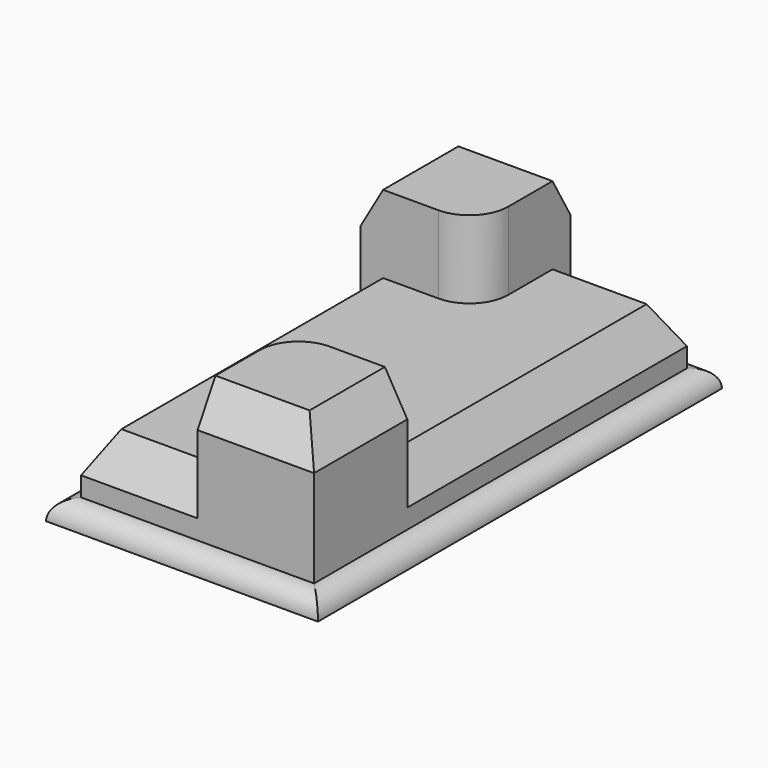
from build123d import *

# Parameters (mm, degrees)
F0_W     = 88.9
F0_H     = 165.1
F1_DEPTH = 6.35
F2_DEPTH = 25.4
F3_DEPTH = 50.8
F4_R     = 6.34999
F5_SIZE2 = 7.3323484187
F5_SIZE  = 12.7
F6_SIZE2 = 7.3323484187
F6_SIZE  = 12.7


# Not quite as in the source:
# - a fillet or chamfer is up to 0.001 mm smaller than in the source, because OpenCascade refuses the exact size


with BuildPart() as f1:
    # F0 (on Top) → F1 (new body)
    with BuildSketch(Plane.XY):
        Rectangle(F0_W, F0_H)
        Polygon((0, 76.2), (38.1, 76.2), (38.1, -38.1), (38.1, -76.2), (0, -76.2), (-38.1, -76.2), (-38.1, 38.1), (-38.1, 76.2), align=None, mode=Mode.SUBTRACT)
    extrude(amount=F1_DEPTH)

    # F0 (on Top) → F2 (join)
    with BuildSketch(Plane.XY):
        with BuildLine():
            Line((38.1, -38.1), (38.1, 76.2))
            Line((38.1, 76.2), (0, 76.2))
            Line((0, 76.2), (0, 50.8))
            ThreePointArc((0, 50.8), (-3.7197438789, 41.8197438789), (-12.7, 38.1))
            Line((-12.7, 38.1), (-38.1, 38.1))
            Line((-38.1, 38.1), (-38.1, -76.2))
            Line((-38.1, -76.2), (0, -76.2))
            Line((0, -76.2), (0, -50.8))
            ThreePointArc((0, -50.8), (3.7197438789, -41.8197438789), (12.7, -38.1))
            Line((12.7, -38.1), (38.1, -38.1))
        make_face()
    extrude(amount=F2_DEPTH)

    # F0 (on Top) → F3 (join)
    with BuildSketch(Plane.XY):
        with BuildLine():
            Line((0, 50.8), (0, 76.2))
            Line((0, 76.2), (-38.1, 76.2))
            Line((-38.1, 76.2), (-38.1, 38.1))
            Line((-38.1, 38.1), (-12.7, 38.1))
            ThreePointArc((-12.7, 38.1), (-3.7197438789, 41.8197438789), (0, 50.8))
        make_face()
        with BuildLine():
            Line((38.1, -76.2), (38.1, -38.1))
            Line((38.1, -38.1), (12.7, -38.1))
            ThreePointArc((12.7, -38.1), (3.7197438789, -41.8197438789), (0, -50.8))
            Line((0, -50.8), (0, -76.2))
            Line((0, -76.2), (38.1, -76.2))
        make_face()
    extrude(amount=F3_DEPTH)

    # F4 (radius 6.35 in the source; OpenCascade refuses exactly that, so slightly less here)
    f4_edges = [f1.edges().sort_by_distance(p)[0] for p in [
        (-44.45, 0, 6.35),
        (0, -82.55, 6.35),
        (44.45, 0, 6.35),
        (0, 82.55, 6.35),
    ]]
    fillet(f4_edges, radius=F4_R)

    # F5
    f5_edges = [f1.edges().sort_by_distance(p)[0] for p in [
        (38.1, 19.05, 25.4),
        (19.05, 76.2, 25.4),
        (-38.1, -19.05, 25.4),
        (-19.05, -76.2, 25.4),
        (19.05, -76.2, 50.8),
        (38.1, -57.15, 50.8),
    ]]
    chamfer(f5_edges, length=F5_SIZE, length2=F5_SIZE2)

    # F6
    f6_edges = [f1.edges().sort_by_distance(p)[0] for p in [
        (-19.05, 76.2, 50.8),
        (-38.1, 57.15, 50.8),
    ]]
    chamfer(f6_edges, length=F6_SIZE, length2=F6_SIZE2)


solid = f1.part
